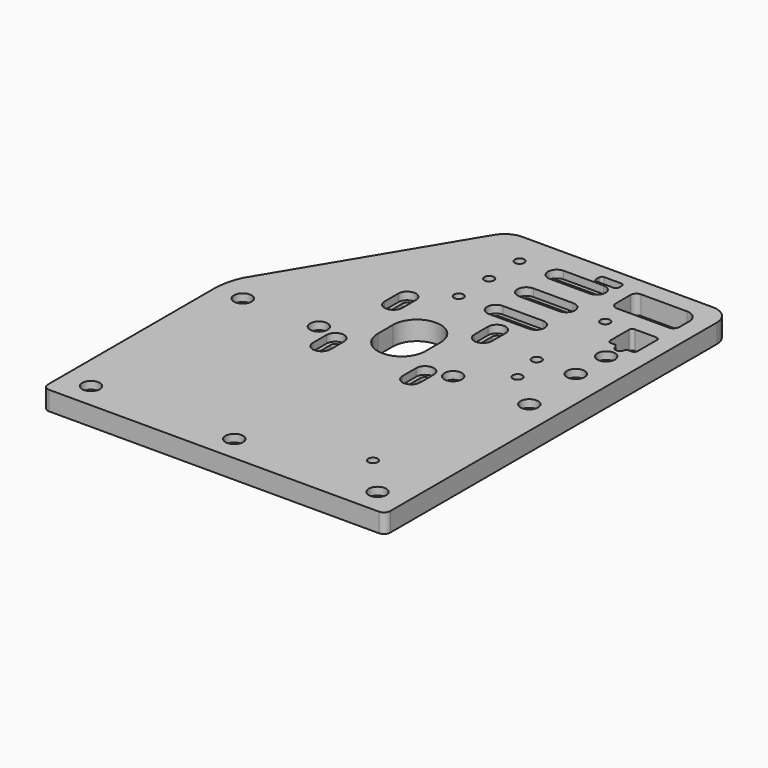
from build123d import *

# Parameters (mm, degrees)
F0_R     = 4.6
F0_R_2   = 2.5
F1_DEPTH = 10
F0_R_3   = 3.6
F2_DEPTH = 6


# Not quite as in the source:
# - ends of sketch curves that miss each other by under 0.0002 mm in the source are joined


with BuildPart() as f1:
    # F0 (on Top) → F1 (new body)
    with BuildSketch(Plane.XY):
        with BuildLine():
            ThreePointArc((-90.000003, -110.40631), (-89.0264648164, -112.7715584011), (-86.6700030006, -113.7661760688))
            Line((-86.6700030006, -113.7661760688), (86.639997, -113.766176))
            ThreePointArc((86.639997, -113.766176), (89.0158757848, -112.7820547848), (89.999997, -110.406176))
            Line((89.999997, -110.406176), (89.999997, 104.053824))
            ThreePointArc((89.999997, 104.053824), (87.1712591943, 110.8980101257), (80.330002, 113.733824))
            Line((80.330002, 113.733824), (-18.849998, 113.733824))
            ThreePointArc((-18.849998, 113.733824), (-25.2573363418, 112.4191498026), (-30.0255163302, 107.9417831984))
            Line((-30.0255163302, 107.9417831984), (-86.679704, 13.65338))
            ThreePointArc((-86.679704, 13.65338), (-89.1601424865, 6.2787905251), (-90.000003, -1.45631))
            Line((-90.000003, -1.45631), (-90.000003, -110.40631))
        make_face()
        with Locations((-75.300003, -100.436176)):
            Circle(F0_R, mode=Mode.SUBTRACT)
        with Locations((-3e-06, -100.436176)):
            Circle(F0_R, mode=Mode.SUBTRACT)
        with Locations((-75.300003, -0.736176)):
            Circle(F0_R, mode=Mode.SUBTRACT)
        with Locations((-35.300003, -0.736176)):
            Circle(F0_R, mode=Mode.SUBTRACT)
        with BuildLine():
            ThreePointArc((-18.930003, -13.556176), (-23.570003, -18.196176), (-28.210003, -13.556176))
            Line((-28.210003, -13.556176), (-28.210003, -4.556176))
            ThreePointArc((-28.210003, -4.556176), (-23.570003, 0.083824), (-18.930003, -4.556176))
            Line((-18.930003, -4.556176), (-18.930003, -13.556176))
        make_face(mode=Mode.SUBTRACT)
        with Locations((75.299997, -100.436176)):
            Circle(F0_R, mode=Mode.SUBTRACT)
        with Locations((56.339997, -79.736176)):
            Circle(F0_R_2, mode=Mode.SUBTRACT)
        with BuildLine():
            ThreePointArc((18.929997, -4.556176), (23.569997, 0.083824), (28.209997, -4.556176))
            Line((28.209997, -4.556176), (28.209997, -13.556176))
            ThreePointArc((28.209997, -13.556176), (23.569997, -18.196176), (18.929997, -13.556176))
            Line((18.929997, -13.556176), (18.929997, -4.556176))
        make_face(mode=Mode.SUBTRACT)
        with Locations((35.299997, -0.736176)):
            Circle(F0_R, mode=Mode.SUBTRACT)
        with Locations((75.299997, -0.736176)):
            Circle(F0_R, mode=Mode.SUBTRACT)
        with BuildLine():
            ThreePointArc((12.499997, 9.513824), (-3e-06, -2.986176), (-12.500003, 9.513824))
            Line((-12.500003, 9.513824), (-12.500003, 19.513824))
            ThreePointArc((-12.500003, 19.513824), (-3e-06, 32.013824), (12.499997, 19.513824))
            Line((12.499997, 19.513824), (12.499997, 9.513824))
        make_face(mode=Mode.SUBTRACT)
        with BuildLine():
            ThreePointArc((-28.210003, 42.583824), (-23.570003, 47.223824), (-18.930003, 42.583824))
            Line((-18.930003, 42.583824), (-18.930003, 33.583824))
            ThreePointArc((-18.930003, 33.583824), (-23.570003, 28.943824), (-28.210003, 33.583824))
            Line((-28.210003, 33.583824), (-28.210003, 42.583824))
        make_face(mode=Mode.SUBTRACT)
        with Locations((-7.310003, 56.173824)):
            Circle(F0_R_2, mode=Mode.SUBTRACT)
        with Locations((-7.310003, 76.173824)):
            Circle(F0_R_2, mode=Mode.SUBTRACT)
        with Locations((-7.310003, 96.173824)):
            Circle(F0_R_2, mode=Mode.SUBTRACT)
        with BuildLine():
            ThreePointArc((28.209997, 33.583824), (23.569997, 28.943824), (18.929997, 33.583824))
            Line((18.929997, 33.583824), (18.929997, 42.583824))
            ThreePointArc((18.929997, 42.583824), (23.569997, 47.223824), (28.209997, 42.583824))
            Line((28.209997, 42.583824), (28.209997, 33.583824))
        make_face(mode=Mode.SUBTRACT)
        with BuildLine():
            ThreePointArc((12.189997, 51.573824), (7.589997, 56.173824), (12.189997, 60.773824))
            Line((12.189997, 60.773824), (33.189997, 60.773824))
            ThreePointArc((33.189997, 60.773824), (37.789997, 56.173824), (33.189997, 51.573824))
            Line((33.189997, 51.573824), (12.189997, 51.573824))
        make_face(mode=Mode.SUBTRACT)
        with Locations((56.339997, 15.263824)):
            Circle(F0_R_2, mode=Mode.SUBTRACT)
        with Locations((52.849997, 32.213824)):
            Circle(F0_R_2, mode=Mode.SUBTRACT)
        with Locations((73.349997, 32.213824)):
            Circle(F0_R, mode=Mode.SUBTRACT)
        with Locations((73.349997, 52.213824)):
            Circle(F0_R, mode=Mode.SUBTRACT)
        with BuildLine():
            ThreePointArc((33.189997, 80.773824), (37.789997, 76.173824), (33.189997, 71.573824))
            Line((33.189997, 71.573824), (12.189997, 71.573824))
            ThreePointArc((12.189997, 71.573824), (7.589997, 76.173824), (12.189997, 80.773824))
            Line((12.189997, 80.773824), (33.189997, 80.773824))
        make_face(mode=Mode.SUBTRACT)
        with BuildLine():
            ThreePointArc((33.189997, 100.773824), (37.789997, 96.173824), (33.189997, 91.573824))
            Line((33.189997, 91.573824), (12.189997, 91.573824))
            ThreePointArc((12.189997, 91.573824), (7.589997, 96.173824), (12.189997, 100.773824))
            Line((12.189997, 100.773824), (33.189997, 100.773824))
        make_face(mode=Mode.SUBTRACT)
        with BuildLine():
            ThreePointArc((28.629997, 101.763824), (27.6117632351, 102.1855902351), (27.189997, 103.203824))
            Line((27.189997, 103.203824), (27.189997, 105.323824))
            ThreePointArc((27.189997, 105.323824), (27.6117632351, 106.3420577649), (28.629997, 106.763824))
            Line((28.629997, 106.763824), (37.749997, 106.763824))
            ThreePointArc((37.749997, 106.763824), (38.7682307649, 106.3420577649), (39.189997, 105.323824))
            Line((39.189997, 105.323824), (39.189997, 103.203824))
            ThreePointArc((39.189997, 103.203824), (38.7682307649, 102.1855902351), (37.749997, 101.763824))
            Line((37.749997, 101.763824), (28.629997, 101.763824))
        make_face(mode=Mode.SUBTRACT)
        with Locations((53.689997, 76.173824)):
            Circle(F0_R_2, mode=Mode.SUBTRACT)
        with BuildLine():
            Line((78.839997, 62.193824), (76.369997, 62.193824))
            Line((76.369997, 62.193824), (75.802984, 61.483539))
            add(Edge.make_bspline(
                [(70.89701, 61.4835398497), (70.8970091503, 59.0305524249), (73.3499965751, 59.030552), (75.802984, 59.0305515751), (75.802984, 61.483539)],
                knots=[3.1415923072, 3.1415923072, 3.1415923072, 4.7123888072, 4.7123888072, 6.2831853072, 6.2831853072, 6.2831853072], degree=2, weights=[1, 0.7071067199, 1, 0.7071067199, 1]))
            Line((70.89701, 61.4835398497), (69.929997, 62.694895))
            Line((69.929997, 62.694895), (67.459997, 62.694895))
            ThreePointArc((67.459997, 62.694895), (66.2861997432, 63.1810977432), (65.799997, 64.354895))
            Line((65.799997, 64.354895), (65.799997, 76.683824))
            ThreePointArc((65.799997, 76.683824), (66.2861997432, 77.8576212568), (67.459997, 78.343824))
            Line((67.459997, 78.343824), (78.839997, 78.343824))
            ThreePointArc((78.839997, 78.343824), (80.0137942568, 77.8576212568), (80.499997, 76.683824))
            Line((80.499997, 76.683824), (80.499997, 63.853824))
            ThreePointArc((80.499997, 63.853824), (80.0137942568, 62.6800267432), (78.839997, 62.193824))
        make_face(mode=Mode.SUBTRACT)
        with BuildLine():
            ThreePointArc((50.139997, 88.263824), (47.9196817071, 89.1835087071), (46.999997, 91.403824))
            Line((46.999997, 91.403824), (46.999997, 101.093824))
            ThreePointArc((46.999997, 101.093824), (47.9196817071, 103.3141392929), (50.139997, 104.233824))
            Line((50.139997, 104.233824), (74.149997, 104.233824))
            ThreePointArc((74.149997, 104.233824), (78.6401250605, 102.3739520605), (80.499997, 97.883824))
            Line((80.499997, 97.883824), (80.499997, 91.403824))
            ThreePointArc((80.499997, 91.403824), (79.5803122929, 89.1835087071), (77.359997, 88.263824))
            Line((77.359997, 88.263824), (50.139997, 88.263824))
        make_face(mode=Mode.SUBTRACT)
    extrude(amount=F1_DEPTH)

    # F0 (on Top) → F2 (join)
    with BuildSketch(Plane.XY):
        with Locations((-75.300003, -100.436176)):
            Circle(F0_R)
        with Locations((-75.300003, -100.436176)):
            Circle(F0_R_3, mode=Mode.SUBTRACT)
        with Locations((-3e-06, -100.436176)):
            Circle(F0_R)
        with Locations((-3e-06, -100.436176)):
            Circle(F0_R_3, mode=Mode.SUBTRACT)
        with Locations((75.299997, -100.436176)):
            Circle(F0_R)
        with Locations((75.299997, -100.436176)):
            Circle(F0_R_3, mode=Mode.SUBTRACT)
        with Locations((75.299997, -0.736176)):
            Circle(F0_R)
        with Locations((75.299997, -0.736176)):
            Circle(F0_R_2, mode=Mode.SUBTRACT)
        with Locations((35.299997, -0.736176)):
            Circle(F0_R)
        with Locations((35.299997, -0.736176)):
            Circle(F0_R_2, mode=Mode.SUBTRACT)
        with Locations((-35.300003, -0.736176)):
            Circle(F0_R)
        with Locations((-35.300003, -0.736176)):
            Circle(F0_R_2, mode=Mode.SUBTRACT)
        with BuildLine():
            Line((-28.210003, -4.556176), (-28.210003, -13.556176))
            ThreePointArc((-28.210003, -13.556176), (-23.570003, -18.196176), (-18.930003, -13.556176))
            Line((-18.930003, -13.556176), (-18.930003, -4.556176))
            ThreePointArc((-18.930003, -4.556176), (-23.570003, 0.083824), (-28.210003, -4.556176))
        make_face()
        with BuildLine():
            ThreePointArc((-21.030003, -13.556176), (-23.570003, -16.096176), (-26.110003, -13.556176))
            Line((-26.110003, -13.556176), (-26.110003, -4.556176))
            ThreePointArc((-26.110003, -4.556176), (-23.570003, -2.016176), (-21.030003, -4.556176))
            Line((-21.030003, -4.556176), (-21.030003, -13.556176))
        make_face(mode=Mode.SUBTRACT)
        with BuildLine():
            Line((-18.930003, 33.583824), (-18.930003, 42.583824))
            ThreePointArc((-18.930003, 42.583824), (-23.570003, 47.223824), (-28.210003, 42.583824))
            Line((-28.210003, 42.583824), (-28.210003, 33.583824))
            ThreePointArc((-28.210003, 33.583824), (-23.570003, 28.943824), (-18.930003, 33.583824))
        make_face()
        with BuildLine():
            ThreePointArc((-21.030003, 33.583824), (-23.570003, 31.043824), (-26.110003, 33.583824))
            Line((-26.110003, 33.583824), (-26.110003, 42.583824))
            ThreePointArc((-26.110003, 42.583824), (-23.570003, 45.123824), (-21.030003, 42.583824))
            Line((-21.030003, 42.583824), (-21.030003, 33.583824))
        make_face(mode=Mode.SUBTRACT)
        with BuildLine():
            Line((18.929997, 42.583824), (18.929997, 33.583824))
            ThreePointArc((18.929997, 33.583824), (23.569997, 28.943824), (28.209997, 33.583824))
            Line((28.209997, 33.583824), (28.209997, 42.583824))
            ThreePointArc((28.209997, 42.583824), (23.569997, 47.223824), (18.929997, 42.583824))
        make_face()
        with BuildLine():
            ThreePointArc((26.109997, 33.583824), (23.569997, 31.043824), (21.029997, 33.583824))
            Line((21.029997, 33.583824), (21.029997, 42.583824))
            ThreePointArc((21.029997, 42.583824), (23.569997, 45.123824), (26.109997, 42.583824))
            Line((26.109997, 42.583824), (26.109997, 33.583824))
        make_face(mode=Mode.SUBTRACT)
        with BuildLine():
            Line((28.209997, -13.556176), (28.209997, -4.556176))
            ThreePointArc((28.209997, -4.556176), (23.569997, 0.083824), (18.929997, -4.556176))
            Line((18.929997, -4.556176), (18.929997, -13.556176))
            ThreePointArc((18.929997, -13.556176), (23.569997, -18.196176), (28.209997, -13.556176))
        make_face()
        with BuildLine():
            ThreePointArc((26.109997, -13.556176), (23.569997, -16.096176), (21.029997, -13.556176))
            Line((21.029997, -13.556176), (21.029997, -4.556176))
            ThreePointArc((21.029997, -4.556176), (23.569997, -2.016176), (26.109997, -4.556176))
            Line((26.109997, -4.556176), (26.109997, -13.556176))
        make_face(mode=Mode.SUBTRACT)
        with Locations((-75.300003, -0.736176)):
            Circle(F0_R)
        with Locations((-75.300003, -0.736176)):
            Circle(F0_R_2, mode=Mode.SUBTRACT)
        with BuildLine():
            Line((12.189997, 71.573824), (33.189997, 71.573824))
            ThreePointArc((33.189997, 71.573824), (37.789997, 76.173824), (33.189997, 80.773824))
            Line((33.189997, 80.773824), (12.189997, 80.773824))
            ThreePointArc((12.189997, 80.773824), (7.589997, 76.173824), (12.189997, 71.573824))
        make_face()
        with BuildLine():
            ThreePointArc((33.189997, 78.673824), (35.689997, 76.173824), (33.189997, 73.673824))
            Line((33.189997, 73.673824), (12.189997, 73.673824))
            ThreePointArc((12.189997, 73.673824), (9.689997, 76.173824), (12.189997, 78.673824))
            Line((12.189997, 78.673824), (33.189997, 78.673824))
        make_face(mode=Mode.SUBTRACT)
        with BuildLine():
            Line((12.189997, 91.573824), (33.189997, 91.573824))
            ThreePointArc((33.189997, 91.573824), (37.789997, 96.173824), (33.189997, 100.773824))
            Line((33.189997, 100.773824), (12.189997, 100.773824))
            ThreePointArc((12.189997, 100.773824), (7.589997, 96.173824), (12.189997, 91.573824))
        make_face()
        with BuildLine():
            ThreePointArc((33.189997, 98.673824), (35.689997, 96.173824), (33.189997, 93.673824))
            Line((33.189997, 93.673824), (12.189997, 93.673824))
            ThreePointArc((12.189997, 93.673824), (9.689997, 96.173824), (12.189997, 98.673824))
            Line((12.189997, 98.673824), (33.189997, 98.673824))
        make_face(mode=Mode.SUBTRACT)
        with BuildLine():
            Line((33.189997, 60.773824), (12.189997, 60.773824))
            ThreePointArc((12.189997, 60.773824), (7.589997, 56.173824), (12.189997, 51.573824))
            Line((12.189997, 51.573824), (33.189997, 51.573824))
            ThreePointArc((33.189997, 51.573824), (37.789997, 56.173824), (33.189997, 60.773824))
        make_face()
        with BuildLine():
            ThreePointArc((33.189997, 58.673824), (35.689997, 56.173824), (33.189997, 53.673824))
            Line((33.189997, 53.673824), (12.189997, 53.673824))
            ThreePointArc((12.189997, 53.673824), (9.689997, 56.173824), (12.189997, 58.673824))
            Line((12.189997, 58.673824), (33.189997, 58.673824))
        make_face(mode=Mode.SUBTRACT)
        with Locations((73.349997, 52.213824)):
            Circle(F0_R)
        with Locations((73.349997, 52.213824)):
            Circle(F0_R_2, mode=Mode.SUBTRACT)
        with Locations((73.349997, 32.213824)):
            Circle(F0_R)
        with Locations((73.349997, 32.213824)):
            Circle(F0_R_2, mode=Mode.SUBTRACT)
    extrude(amount=F2_DEPTH)


solid = f1.part
